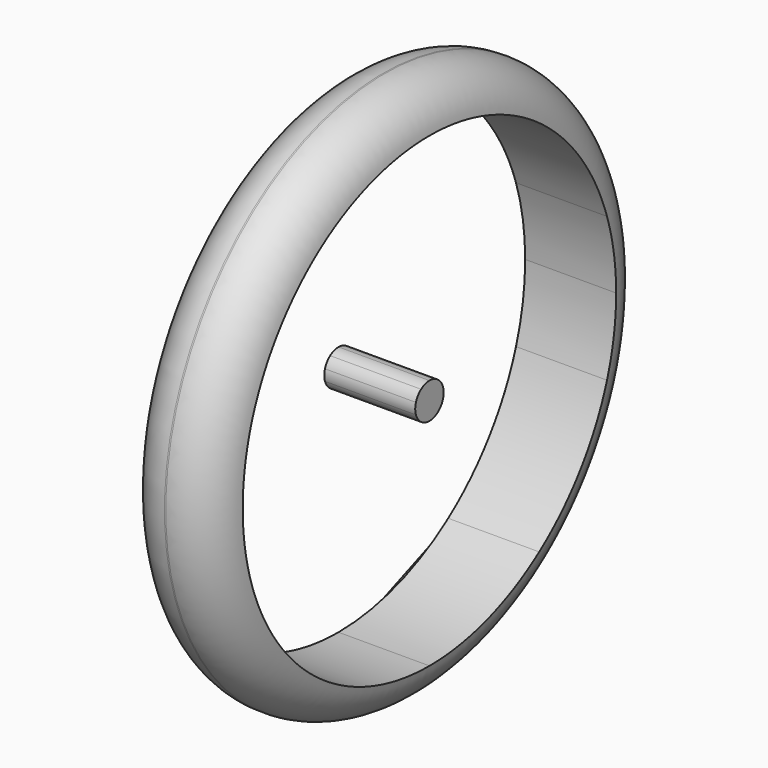
from build123d import *

# Parameters (mm, degrees)
F0_R     = 76.3818717889
F3_DEPTH = 25.4
F4_DEPTH = 25.4


# Not quite as in the source:
# - a fillet or chamfer that OpenCascade refuses, or shapes differently, is made with other operations: its cross-section is extruded or revolved along the edge and cut away or added
# - the program builds the solid bodies; features that only make, move or delete a surface that nothing else refers to are left out


with BuildPart() as f3:
    # F0 (on Right) → F3 (new body)
    with BuildSketch(Plane.YZ):
        Circle(F0_R)
        with BuildLine():
            ThreePointArc((61.9708271601, 20.1355423362), (64.3577562368, 10.1932672021), (65.1599837637, 0))
            ThreePointArc((65.1599837637, 0), (64.3577562368, -10.1932672021), (61.9708271601, -20.1355423362))
            ThreePointArc((61.9708271601, -20.1355423362), (52.715534218, -38.3000774959), (38.3000774959, -52.715534218))
            ThreePointArc((38.3000774959, -52.715534218), (20.1355423362, -61.9708271601), (0, -65.1599837637))
            ThreePointArc((0, -65.1599837637), (-20.1355423362, -61.9708271601), (-38.3000774959, -52.715534218))
            ThreePointArc((-38.3000774959, -52.715534218), (-52.715534218, -38.3000774959), (-61.9708271601, -20.1355423362))
            ThreePointArc((-61.9708271601, -20.1355423362), (-65.1599837637, 0), (-61.9708271601, 20.1355423362))
            ThreePointArc((-61.9708271601, 20.1355423362), (-52.715534218, 38.3000774959), (-38.3000774959, 52.715534218))
            ThreePointArc((-38.3000774959, 52.715534218), (-20.1355423362, 61.9708271601), (0, 65.1599837637))
            ThreePointArc((0, 65.1599837637), (20.1355423362, 61.9708271601), (38.3000774959, 52.715534218))
            ThreePointArc((38.3000774959, 52.715534218), (52.715534218, 38.3000774959), (61.9708271601, 20.1355423362))
        make_face(mode=Mode.SUBTRACT)
    extrude(amount=F3_DEPTH)

    # F5: fillet of radius 12.7 on 1 edges, made by hand

    # F5_s1 → F5_t2 (revolve, cut)
    with BuildSketch(Plane.XY):
        with BuildLine():
            ThreePointArc((12.7854505187, 76.3822717889), (21.2275412664, 73.1706792347), (25.4003972784, 65.1600303453))
            Line((25.4003972784, 65.1600303453), (26.6618919544, 65.3079427695))
            ThreePointArc((26.6618919544, 65.3079427695), (26.6701365685, 70.7709510671), (26.6701365685, 76.3818717889))
            Line((26.6701365685, 76.3818717889), (25.4, 77.6520083575))
            ThreePointArc((25.4, 77.6520083575), (19.0927252593, 77.6520083575), (12.7854505187, 77.6524083575))
            Line((12.7854505187, 77.6524083575), (12.7854505187, 76.3822717889))
        make_face()
    revolve(axis=Axis((25.4, 0, 0), (1, 0, 0)), mode=Mode.SUBTRACT)

    # F6: fillet of radius 12.7 on 3 edges, made by hand

    # F6_s1 → F6_t2 (revolve, cut)
    with BuildSketch(Plane.XY):
        with BuildLine():
            ThreePointArc((12.6145494813, 76.3822717889), (4.1724587336, 73.1706792347), (-0.0003972784, 65.1600303453))
            Line((-0.0003972784, 65.1600303453), (-1.2618919544, 65.3079427695))
            ThreePointArc((-1.2618919544, 65.3079427695), (-1.2701365685, 70.7709510671), (-1.2701365685, 76.3818717889))
            Line((-1.2701365685, 76.3818717889), (0, 77.6520083575))
            ThreePointArc((0, 77.6520083575), (6.3072747407, 77.6520083575), (12.6145494813, 77.6524083575))
            Line((12.6145494813, 77.6524083575), (12.6145494813, 76.3822717889))
        make_face()
    revolve(axis=Axis((0, 0, 0), (1, 0, 0)), mode=Mode.SUBTRACT)


with BuildPart() as f4:
    # F0 (on Right) → F4 (new body)
    with BuildSketch(Plane.YZ):
        with BuildLine():
            ThreePointArc((4.9653046516, 0), (4.9041735119, 0.7767447769), (4.7222853443, 1.5343635196))
            ThreePointArc((4.7222853443, 1.5343635196), (4.0170158454, 2.9185328474), (2.9185328474, 4.0170158454))
            ThreePointArc((2.9185328474, 4.0170158454), (1.5343635196, 4.7222853443), (0, 4.9653046516))
            ThreePointArc((0, 4.9653046516), (-1.5343635196, 4.7222853443), (-2.9185328474, 4.0170158454))
            ThreePointArc((-2.9185328474, 4.0170158454), (-4.0170158454, 2.9185328474), (-4.7222853443, 1.5343635196))
            ThreePointArc((-4.7222853443, 1.5343635196), (-4.9653046516, 0), (-4.7222853443, -1.5343635196))
            ThreePointArc((-4.7222853443, -1.5343635196), (-4.0170158454, -2.9185328474), (-2.9185328474, -4.0170158454))
            ThreePointArc((-2.9185328474, -4.0170158454), (-1.5343635196, -4.7222853443), (0, -4.9653046516))
            ThreePointArc((0, -4.9653046516), (1.5343635196, -4.7222853443), (2.9185328474, -4.0170158454))
            ThreePointArc((2.9185328474, -4.0170158454), (4.0170158454, -2.9185328474), (4.7222853443, -1.5343635196))
            ThreePointArc((4.7222853443, -1.5343635196), (4.9041735119, -0.7767447769), (4.9653046516, 0))
        make_face()
    extrude(amount=F4_DEPTH)


solid = Compound([f3.part, f4.part])
